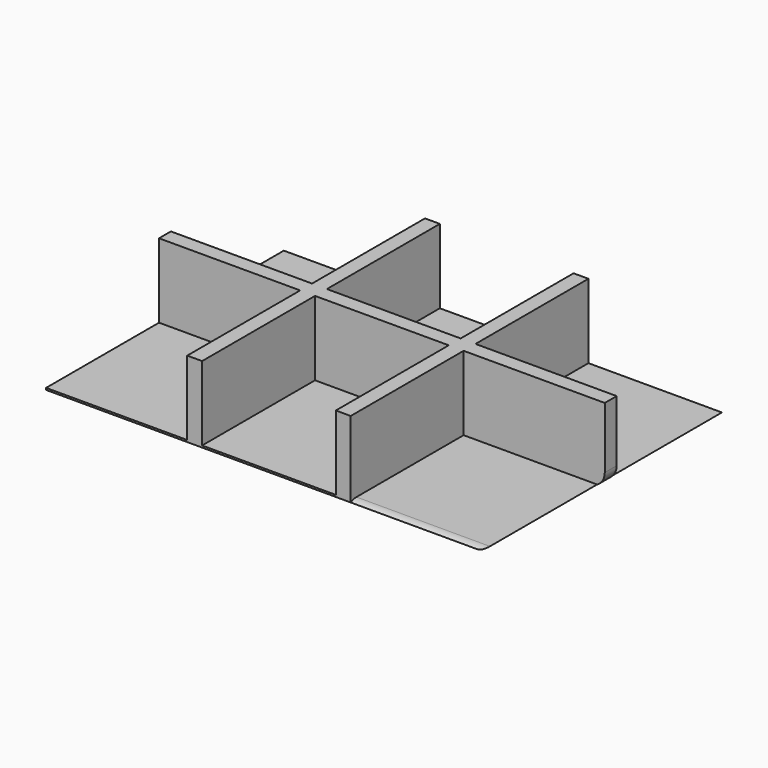
from build123d import *

# Parameters (mm, degrees)
F0_W         = 50.8
F0_H         = 50.8
F16_DEPTH    = 0.635
F13_E4_W     = 50.8
F13_E4_H     = 25.4
F17_DEPTH    = 2.54
F11_E6_W     = 50.8
F11_E6_H     = 25.4
F11_E5_W     = 50.8
F11_E5_H     = 25.4
F18_DEPTH    = 2.54
F9_E0_W      = 25.4
F9_E0_H      = 25.4
F9_E3_W      = 25.4
F9_E3_H      = 25.4
F19_DEPTH    = 2.54
F7_E7_W      = 50.8
F7_E7_H      = 25.4
F20_DEPTH    = 2.54
F3_E1_W      = 50.8
F3_E1_H      = 25.4
F21_DEPTH    = 2.54
F1_E2_W      = 50.8
F1_E2_H      = 25.4
F22_DEPTH    = 2.54
F23_R        = 5.08
F24_T1_DEPTH = 51.7877054869


# Not quite as in the source:
# - a fillet or chamfer that OpenCascade refuses, or shapes differently, is made with other operations: its cross-section is extruded or revolved along the edge and cut away or added
# - the program builds the solid bodies; features that only make, move or delete a surface that nothing else refers to are left out


with BuildPart() as f16:
    # F0 (on Top) → F16 (new body)
    with BuildSketch(Plane.XY):
        Polygon((-25.4, 0), (0, 0), (25.4, 0), (25.4, 50.8), (-25.4, 50.8), align=None)
        Polygon((25.4, 0), (0, 0), (-25.4, 0), (-25.4, -50.8), (25.4, -50.8), align=None)
        with Locations((50.8, -25.4)):
            Rectangle(F0_W, F0_H)
        with Locations((50.8, 25.4)):
            Rectangle(F0_W, F0_H)
        with Locations((-50.8, -25.4)):
            Rectangle(F0_W, F0_H)
        with Locations((-50.8, 25.4)):
            Rectangle(F0_W, F0_H)
    extrude(amount=-F16_DEPTH)

    # F13_E4 (on explicit) → F17 (join, symmetric)
    with BuildSketch(Plane(origin=(-25.4, 0, 0), x_dir=(-1, 0, 0), z_dir=(0, 1, 0))):
        with Locations((25.4, 12.7)):
            Rectangle(F13_E4_W, F13_E4_H)
    extrude(amount=F17_DEPTH, both=True)

    # F11_E6 (on explicit) + F11_E5 (on explicit) → F18 (join, symmetric)
    with BuildSketch(Plane.YZ.offset(-25.4)):
        with Locations((25.4, 12.7)):
            Rectangle(F11_E6_W, F11_E6_H)
    with BuildSketch(Plane(origin=(-25.4, 0, 0), x_dir=(0, -1, 0), z_dir=(-1, 0, 0))):
        with Locations((25.4, 12.7)):
            Rectangle(F11_E5_W, F11_E5_H)
    extrude(amount=F18_DEPTH, both=True, dir=(1, 0, 0))

    # F9_E0 (on explicit) + F9_E3 (on explicit) → F19 (join, symmetric)
    with BuildSketch(Plane.XZ):
        with Locations((12.7, 12.7)):
            Rectangle(F9_E0_W, F9_E0_H)
    with BuildSketch(Plane(origin=(0, 0, 0), x_dir=(-1, 0, 0), z_dir=(0, 1, 0))):
        with Locations((12.7, 12.7)):
            Rectangle(F9_E3_W, F9_E3_H)
    extrude(amount=F19_DEPTH, both=True, dir=(0, -1, 0))

    # F7_E7 (on explicit) → F20 (join, symmetric)
    with BuildSketch(Plane.YZ.offset(25.4)):
        with Locations((25.4, 12.7)):
            Rectangle(F7_E7_W, F7_E7_H)
    extrude(amount=F20_DEPTH, both=True)

    # F3_E1 (on explicit) → F21 (join, symmetric)
    with BuildSketch(Plane(origin=(25.4, 0, 0), x_dir=(0, -1, 0), z_dir=(-1, 0, 0))):
        with Locations((25.4, 12.7)):
            Rectangle(F3_E1_W, F3_E1_H)
    extrude(amount=F21_DEPTH, both=True)

    # F1_E2 (on explicit) → F22 (join, symmetric)
    with BuildSketch(Plane(origin=(25.4, 0, 0), x_dir=(1, 0, 0), z_dir=(0, -1, 0))):
        with Locations((25.4, 12.7)):
            Rectangle(F1_E2_W, F1_E2_H)
    extrude(amount=F22_DEPTH, both=True)

    # F23
    f23_edges = [f16.edges().sort_by_distance(p)[0] for p in [
        (76.2, 0, -0.635),
    ]]
    fillet(f23_edges, radius=F23_R)

    # F24: fillet of radius 5.08 on 1 edges, made by hand

    # F24_s2 → F24_t1 (cut)
    with BuildSketch(Plane.YZ.offset(27.94)):
        with BuildLine():
            ThreePointArc((-50.8, -0.635), (-49.6106555752, -0.1613111503), (-48.3406555752, 0))
            Line((-48.3406555752, 0), (-50.8, 0))
            Line((-50.8, 0), (-50.8, -0.635))
        make_face()
    extrude(amount=F24_T1_DEPTH, mode=Mode.SUBTRACT)


solid = f16.part
